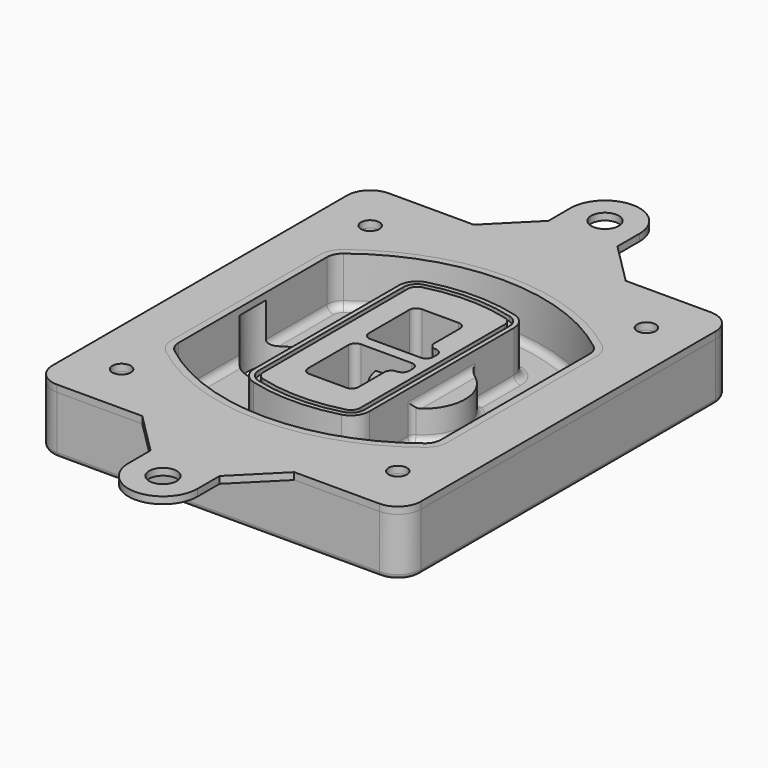
from build123d import *

# Parameters (mm, degrees)
F0_R      = 4
F1_DEPTH  = 25
F2_DEPTH  = 3
F3_DEPTH  = 18
F5_DEPTH  = 21
F6_DEPTH  = 2
F8_DEPTH  = 20
F9_DEPTH  = 16
F10_DEPTH = 25
F7_R      = 6
F7_R_2    = 4
F11_DEPTH = 6
F13_DEPTH = 9
F14_R     = 3
F15_R     = 2
F16_R     = 6
F16_R_2   = 4
F17_DEPTH = 3


# Not quite as in the source:
# - a feature names something its author has since deleted; it is built from what else it names


with BuildPart() as f1:
    # F0 (on Top) → F1 (new body)
    with BuildSketch(Plane.XY):
        with BuildLine():
            ThreePointArc((-80, -80), (-77.0710678119, -87.0710678119), (-70, -90))
            Line((-70, -90), (70, -90))
            ThreePointArc((70, -90), (77.0710678119, -87.0710678119), (80, -80))
            Line((80, -80), (80, 80))
            ThreePointArc((80, 80), (77.0710678119, 87.0710678119), (70, 90))
            Line((70, 90), (-70, 90))
            ThreePointArc((-70, 90), (-77.0710678119, 87.0710678119), (-80, 80))
            Line((-80, 80), (-80, -80))
        make_face()
        with Locations((-60, -67.5)):
            Circle(F0_R, mode=Mode.SUBTRACT)
        with Locations((60, -67.5)):
            Circle(F0_R, mode=Mode.SUBTRACT)
        with Locations((-60, 67.5)):
            Circle(F0_R, mode=Mode.SUBTRACT)
        with BuildLine():
            ThreePointArc((-64, 40.2934422872), (-62.5820384798, 46.4328484224), (-58.6153846154, 51.3286200352))
            ThreePointArc((-58.6153846154, 51.3286200352), (0, 71.5), (58.6153846154, 51.3286200352))
            ThreePointArc((58.6153846154, 51.3286200352), (62.5820384798, 46.4328484224), (64, 40.2934422872))
            Line((64, 40.2934422872), (64, -40.2934422872))
            ThreePointArc((64, -40.2934422872), (62.5820384798, -46.4328484224), (58.6153846154, -51.3286200352))
            ThreePointArc((58.6153846154, -51.3286200352), (0, -71.5), (-58.6153846154, -51.3286200352))
            ThreePointArc((-58.6153846154, -51.3286200352), (-62.5820384798, -46.4328484224), (-64, -40.2934422872))
            Line((-64, -40.2934422872), (-64, 40.2934422872))
        make_face(mode=Mode.SUBTRACT)
        with Locations((60, 67.5)):
            Circle(F0_R, mode=Mode.SUBTRACT)
        with BuildLine():
            ThreePointArc((58.6153846154, 51.3286200352), (0, 71.5), (-58.6153846154, 51.3286200352))
            ThreePointArc((-58.6153846154, 51.3286200352), (-62.5820384798, 46.4328484224), (-64, 40.2934422872))
            Line((-64, 40.2934422872), (-64, -40.2934422872))
            ThreePointArc((-64, -40.2934422872), (-62.5820384798, -46.4328484224), (-58.6153846154, -51.3286200352))
            ThreePointArc((-58.6153846154, -51.3286200352), (0, -71.5), (58.6153846154, -51.3286200352))
            ThreePointArc((58.6153846154, -51.3286200352), (62.5820384798, -46.4328484224), (64, -40.2934422872))
            Line((64, -40.2934422872), (64, 40.2934422872))
            ThreePointArc((64, 40.2934422872), (62.5820384798, 46.4328484224), (58.6153846154, 51.3286200352))
        make_face()
        with BuildLine():
            Line((-60, -40.2934422872), (-60, 40.2934422872))
            ThreePointArc((-60, 40.2934422872), (-58.9871703427, 44.6787323838), (-56.1538461538, 48.1757121072))
            ThreePointArc((-56.1538461538, 48.1757121072), (0, 67.5), (56.1538461538, 48.1757121072))
            ThreePointArc((56.1538461538, 48.1757121072), (58.9871703427, 44.6787323838), (60, 40.2934422872))
            Line((60, 40.2934422872), (60, -40.2934422872))
            ThreePointArc((60, -40.2934422872), (58.9871703427, -44.6787323838), (56.1538461538, -48.1757121072))
            ThreePointArc((56.1538461538, -48.1757121072), (0, -67.5), (-56.1538461538, -48.1757121072))
            ThreePointArc((-56.1538461538, -48.1757121072), (-58.9871703427, -44.6787323838), (-60, -40.2934422872))
        make_face(mode=Mode.SUBTRACT)
        with BuildLine():
            ThreePointArc((-56.1538461538, 48.1757121072), (-58.9871703427, 44.6787323838), (-60, 40.2934422872))
            Line((-60, 40.2934422872), (-60, -40.2934422872))
            ThreePointArc((-60, -40.2934422872), (-58.9871703427, -44.6787323838), (-56.1538461538, -48.1757121072))
            ThreePointArc((-56.1538461538, -48.1757121072), (0, -67.5), (56.1538461538, -48.1757121072))
            ThreePointArc((56.1538461538, -48.1757121072), (58.9871703427, -44.6787323838), (60, -40.2934422872))
            Line((60, -40.2934422872), (60, 40.2934422872))
            ThreePointArc((60, 40.2934422872), (58.9871703427, 44.6787323838), (56.1538461538, 48.1757121072))
            ThreePointArc((56.1538461538, 48.1757121072), (0, 67.5), (-56.1538461538, 48.1757121072))
        make_face()
        with BuildLine():
            ThreePointArc((54.3076923077, 45.8110311612), (56.2910192399, 43.3631453548), (57, 40.2934422872))
            Line((57, 40.2934422872), (57, -40.2934422872))
            ThreePointArc((57, -40.2934422872), (56.2910192399, -43.3631453548), (54.3076923077, -45.8110311612))
            ThreePointArc((54.3076923077, -45.8110311612), (0, -64.5), (-54.3076923077, -45.8110311612))
            ThreePointArc((-54.3076923077, -45.8110311612), (-56.2910192399, -43.3631453548), (-57, -40.2934422872))
            Line((-57, -40.2934422872), (-57, 40.2934422872))
            ThreePointArc((-57, 40.2934422872), (-56.2910192399, 43.3631453548), (-54.3076923077, 45.8110311612))
            ThreePointArc((-54.3076923077, 45.8110311612), (0, 64.5), (54.3076923077, 45.8110311612))
        make_face(mode=Mode.SUBTRACT)
        with BuildLine():
            Line((57, -40.2934422872), (57, 40.2934422872))
            ThreePointArc((57, 40.2934422872), (56.2910192399, 43.3631453548), (54.3076923077, 45.8110311612))
            ThreePointArc((54.3076923077, 45.8110311612), (0, 64.5), (-54.3076923077, 45.8110311612))
            ThreePointArc((-54.3076923077, 45.8110311612), (-56.2910192399, 43.3631453548), (-57, 40.2934422872))
            Line((-57, 40.2934422872), (-57, -40.2934422872))
            ThreePointArc((-57, -40.2934422872), (-56.2910192399, -43.3631453548), (-54.3076923077, -45.8110311612))
            ThreePointArc((-54.3076923077, -45.8110311612), (0, -64.5), (54.3076923077, -45.8110311612))
            ThreePointArc((54.3076923077, -45.8110311612), (56.2910192399, -43.3631453548), (57, -40.2934422872))
        make_face()
    extrude(amount=-F1_DEPTH)

    # F0 (on Top) → F2 (join)
    with BuildSketch(Plane.XY):
        with BuildLine():
            ThreePointArc((-56.1538461538, 48.1757121072), (-58.9871703427, 44.6787323838), (-60, 40.2934422872))
            Line((-60, 40.2934422872), (-60, -40.2934422872))
            ThreePointArc((-60, -40.2934422872), (-58.9871703427, -44.6787323838), (-56.1538461538, -48.1757121072))
            ThreePointArc((-56.1538461538, -48.1757121072), (0, -67.5), (56.1538461538, -48.1757121072))
            ThreePointArc((56.1538461538, -48.1757121072), (58.9871703427, -44.6787323838), (60, -40.2934422872))
            Line((60, -40.2934422872), (60, 40.2934422872))
            ThreePointArc((60, 40.2934422872), (58.9871703427, 44.6787323838), (56.1538461538, 48.1757121072))
            ThreePointArc((56.1538461538, 48.1757121072), (0, 67.5), (-56.1538461538, 48.1757121072))
        make_face()
        with BuildLine():
            ThreePointArc((54.3076923077, 45.8110311612), (56.2910192399, 43.3631453548), (57, 40.2934422872))
            Line((57, 40.2934422872), (57, -40.2934422872))
            ThreePointArc((57, -40.2934422872), (56.2910192399, -43.3631453548), (54.3076923077, -45.8110311612))
            ThreePointArc((54.3076923077, -45.8110311612), (0, -64.5), (-54.3076923077, -45.8110311612))
            ThreePointArc((-54.3076923077, -45.8110311612), (-56.2910192399, -43.3631453548), (-57, -40.2934422872))
            Line((-57, -40.2934422872), (-57, 40.2934422872))
            ThreePointArc((-57, 40.2934422872), (-56.2910192399, 43.3631453548), (-54.3076923077, 45.8110311612))
            ThreePointArc((-54.3076923077, 45.8110311612), (0, 64.5), (54.3076923077, 45.8110311612))
        make_face(mode=Mode.SUBTRACT)
    extrude(amount=F2_DEPTH)

    # F0 (on Top) → F3 (cut)
    with BuildSketch(Plane.XY):
        with BuildLine():
            Line((57, -40.2934422872), (57, 40.2934422872))
            ThreePointArc((57, 40.2934422872), (56.2910192399, 43.3631453548), (54.3076923077, 45.8110311612))
            ThreePointArc((54.3076923077, 45.8110311612), (0, 64.5), (-54.3076923077, 45.8110311612))
            ThreePointArc((-54.3076923077, 45.8110311612), (-56.2910192399, 43.3631453548), (-57, 40.2934422872))
            Line((-57, 40.2934422872), (-57, -40.2934422872))
            ThreePointArc((-57, -40.2934422872), (-56.2910192399, -43.3631453548), (-54.3076923077, -45.8110311612))
            ThreePointArc((-54.3076923077, -45.8110311612), (0, -64.5), (54.3076923077, -45.8110311612))
            ThreePointArc((54.3076923077, -45.8110311612), (56.2910192399, -43.3631453548), (57, -40.2934422872))
        make_face()
    extrude(amount=-F3_DEPTH, mode=Mode.SUBTRACT)

    # F4 (on face) → F5 (join, through all)
    with BuildSketch(Plane.XY.offset(3)):
        with BuildLine():
            ThreePointArc((-25, -39.2465276821), (-23.3511545998, -44.1109737193), (-19.0842911877, -46.9702398883))
            ThreePointArc((-19.0842911877, -46.9702398883), (0, -49.5), (19.0842911877, -46.9702398883))
            ThreePointArc((19.0842911877, -46.9702398883), (23.3511545998, -44.1109737193), (25, -39.2465276821))
            Line((25, -39.2465276821), (25, 39.2465276821))
            ThreePointArc((25, 39.2465276821), (23.3511545998, 44.1109737193), (19.0842911877, 46.9702398883))
            ThreePointArc((19.0842911877, 46.9702398883), (0, 49.5), (-19.0842911877, 46.9702398883))
            ThreePointArc((-19.0842911877, 46.9702398883), (-23.3511545998, 44.1109737193), (-25, 39.2465276821))
            Line((-25, 39.2465276821), (-25, -39.2465276821))
        make_face()
        with BuildLine():
            ThreePointArc((18.5632183908, 45.0393118368), (21.7633659499, 42.89486221), (23, 39.2465276821))
            Line((23, 39.2465276821), (23, -39.2465276821))
            ThreePointArc((23, -39.2465276821), (21.7633659499, -42.89486221), (18.5632183908, -45.0393118368))
            ThreePointArc((18.5632183908, -45.0393118368), (0, -47.5), (-18.5632183908, -45.0393118368))
            ThreePointArc((-18.5632183908, -45.0393118368), (-21.7633659499, -42.89486221), (-23, -39.2465276821))
            Line((-23, -39.2465276821), (-23, 39.2465276821))
            ThreePointArc((-23, 39.2465276821), (-21.7633659499, 42.89486221), (-18.5632183908, 45.0393118368))
            ThreePointArc((-18.5632183908, 45.0393118368), (0, 47.5), (18.5632183908, 45.0393118368))
        make_face(mode=Mode.SUBTRACT)
        with BuildLine():
            Line((23, -39.2465276821), (23, 39.2465276821))
            ThreePointArc((23, 39.2465276821), (21.7633659499, 42.89486221), (18.5632183908, 45.0393118368))
            ThreePointArc((18.5632183908, 45.0393118368), (0, 47.5), (-18.5632183908, 45.0393118368))
            ThreePointArc((-18.5632183908, 45.0393118368), (-21.7633659499, 42.89486221), (-23, 39.2465276821))
            Line((-23, 39.2465276821), (-23, -39.2465276821))
            ThreePointArc((-23, -39.2465276821), (-21.7633659499, -42.89486221), (-18.5632183908, -45.0393118368))
            ThreePointArc((-18.5632183908, -45.0393118368), (0, -47.5), (18.5632183908, -45.0393118368))
            ThreePointArc((18.5632183908, -45.0393118368), (21.7633659499, -42.89486221), (23, -39.2465276821))
        make_face()
        with BuildLine():
            ThreePointArc((18.0421455939, 43.1083837852), (20.1755772999, 41.6787507007), (21, 39.2465276821))
            Line((21, 39.2465276821), (21, -39.2465276821))
            ThreePointArc((21, -39.2465276821), (20.1755772999, -41.6787507007), (18.0421455939, -43.1083837852))
            ThreePointArc((18.0421455939, -43.1083837852), (0, -45.5), (-18.0421455939, -43.1083837852))
            ThreePointArc((-18.0421455939, -43.1083837852), (-20.1755772999, -41.6787507007), (-21, -39.2465276821))
            Line((-21, -39.2465276821), (-21, 39.2465276821))
            ThreePointArc((-21, 39.2465276821), (-20.1755772999, 41.6787507007), (-18.0421455939, 43.1083837852))
            ThreePointArc((-18.0421455939, 43.1083837852), (0, 45.5), (18.0421455939, 43.1083837852))
        make_face(mode=Mode.SUBTRACT)
        with BuildLine():
            Line((21, -39.2465276821), (21, 39.2465276821))
            ThreePointArc((21, 39.2465276821), (20.1755772999, 41.6787507007), (18.0421455939, 43.1083837852))
            ThreePointArc((18.0421455939, 43.1083837852), (0, 45.5), (-18.0421455939, 43.1083837852))
            ThreePointArc((-18.0421455939, 43.1083837852), (-20.1755772999, 41.6787507007), (-21, 39.2465276821))
            Line((-21, 39.2465276821), (-21, -39.2465276821))
            ThreePointArc((-21, -39.2465276821), (-20.1755772999, -41.6787507007), (-18.0421455939, -43.1083837852))
            ThreePointArc((-18.0421455939, -43.1083837852), (0, -45.5), (18.0421455939, -43.1083837852))
            ThreePointArc((18.0421455939, -43.1083837852), (20.1755772999, -41.6787507007), (21, -39.2465276821))
        make_face()
        with BuildLine():
            Line((-8, -2.5), (14, -2.5))
            ThreePointArc((14, -2.5), (16.1213203436, -3.3786796564), (17, -5.5))
            Line((17, -5.5), (17, -7.5))
            ThreePointArc((17, -7.5), (16.1213203436, -9.6213203436), (14, -10.5))
            ThreePointArc((14, -10.5), (11.8786796564, -11.3786796564), (11, -13.5))
            Line((11, -13.5), (11, -27.5))
            ThreePointArc((11, -27.5), (10.1213203436, -29.6213203436), (8, -30.5))
            Line((8, -30.5), (-8, -30.5))
            ThreePointArc((-8, -30.5), (-10.1213203436, -29.6213203436), (-11, -27.5))
            Line((-11, -27.5), (-11, -5.5))
            ThreePointArc((-11, -5.5), (-10.1213203436, -3.3786796564), (-8, -2.5))
        make_face(mode=Mode.SUBTRACT)
        with BuildLine():
            ThreePointArc((-8, 2.5), (-10.1213203436, 3.3786796564), (-11, 5.5))
            Line((-11, 5.5), (-11, 27.5))
            ThreePointArc((-11, 27.5), (-10.1213203436, 29.6213203436), (-8, 30.5))
            Line((-8, 30.5), (8, 30.5))
            ThreePointArc((8, 30.5), (10.1213203436, 29.6213203436), (11, 27.5))
            Line((11, 27.5), (11, 13.5))
            ThreePointArc((11, 13.5), (11.8786796564, 11.3786796564), (14, 10.5))
            ThreePointArc((14, 10.5), (16.1213203436, 9.6213203436), (17, 7.5))
            Line((17, 7.5), (17, 5.5))
            ThreePointArc((17, 5.5), (16.1213203436, 3.3786796564), (14, 2.5))
            Line((14, 2.5), (-8, 2.5))
        make_face(mode=Mode.SUBTRACT)
    extrude(amount=-F5_DEPTH)

    # F4 (on face) → F6 (cut)
    with BuildSketch(Plane.XY.offset(3)):
        with BuildLine():
            Line((23, -39.2465276821), (23, 39.2465276821))
            ThreePointArc((23, 39.2465276821), (21.7633659499, 42.89486221), (18.5632183908, 45.0393118368))
            ThreePointArc((18.5632183908, 45.0393118368), (0, 47.5), (-18.5632183908, 45.0393118368))
            ThreePointArc((-18.5632183908, 45.0393118368), (-21.7633659499, 42.89486221), (-23, 39.2465276821))
            Line((-23, 39.2465276821), (-23, -39.2465276821))
            ThreePointArc((-23, -39.2465276821), (-21.7633659499, -42.89486221), (-18.5632183908, -45.0393118368))
            ThreePointArc((-18.5632183908, -45.0393118368), (0, -47.5), (18.5632183908, -45.0393118368))
            ThreePointArc((18.5632183908, -45.0393118368), (21.7633659499, -42.89486221), (23, -39.2465276821))
        make_face()
        with BuildLine():
            ThreePointArc((18.0421455939, 43.1083837852), (20.1755772999, 41.6787507007), (21, 39.2465276821))
            Line((21, 39.2465276821), (21, -39.2465276821))
            ThreePointArc((21, -39.2465276821), (20.1755772999, -41.6787507007), (18.0421455939, -43.1083837852))
            ThreePointArc((18.0421455939, -43.1083837852), (0, -45.5), (-18.0421455939, -43.1083837852))
            ThreePointArc((-18.0421455939, -43.1083837852), (-20.1755772999, -41.6787507007), (-21, -39.2465276821))
            Line((-21, -39.2465276821), (-21, 39.2465276821))
            ThreePointArc((-21, 39.2465276821), (-20.1755772999, 41.6787507007), (-18.0421455939, 43.1083837852))
            ThreePointArc((-18.0421455939, 43.1083837852), (0, 45.5), (18.0421455939, 43.1083837852))
        make_face(mode=Mode.SUBTRACT)
    extrude(amount=-F6_DEPTH, mode=Mode.SUBTRACT)

    # F7 (on face) → F8 (join)
    with BuildSketch(Plane(origin=(0, 0, -25), x_dir=(1, 0, 0), z_dir=(0, 0, -1))):
        with BuildLine():
            ThreePointArc((3.28842436, 0), (16.7567035675, 13.4682792075), (30.224982775, 0))
            Line((30.224982775, 0), (35.224982775, 0))
            ThreePointArc((35.224982775, 0), (16.7567035675, 18.4682792075), (-1.71157564, 0))
            Line((-1.71157564, 0), (3.28842436, 0))
        make_face()
        with BuildLine():
            Line((3.28842436, 0), (30.224982775, 0))
            ThreePointArc((30.224982775, 0), (16.7567035675, 13.4682792075), (3.28842436, 0))
        make_face()
        with BuildLine():
            ThreePointArc((3.28842436, 0), (16.7567035675, -13.4682792075), (30.224982775, 0))
            Line((30.224982775, 0), (3.28842436, 0))
        make_face()
        with BuildLine():
            Line((35.224982775, 0), (30.224982775, 0))
            ThreePointArc((30.224982775, 0), (16.7567035675, -13.4682792075), (3.28842436, 0))
            Line((3.28842436, 0), (-1.71157564, 0))
            ThreePointArc((-1.71157564, 0), (16.7567035675, -18.4682792075), (35.224982775, 0))
        make_face()
    extrude(amount=-F8_DEPTH)

    # F7 (on face) → F9 (cut)
    with BuildSketch(Plane(origin=(0, 0, -25), x_dir=(1, 0, 0), z_dir=(0, 0, -1))):
        with BuildLine():
            Line((3.28842436, 0), (30.224982775, 0))
            ThreePointArc((30.224982775, 0), (16.7567035675, 13.4682792075), (3.28842436, 0))
        make_face()
        with BuildLine():
            ThreePointArc((3.28842436, 0), (16.7567035675, -13.4682792075), (30.224982775, 0))
            Line((30.224982775, 0), (3.28842436, 0))
        make_face()
    extrude(amount=-F9_DEPTH, mode=Mode.SUBTRACT)

    # F7 (on face) → F10 (cut)
    with BuildSketch(Plane(origin=(0, 0, -25), x_dir=(1, 0, 0), z_dir=(0, 0, -1))):
        with BuildLine():
            Line((-59.0318229325, 0), (-32.0952645175, 0))
            ThreePointArc((-32.0952645175, 0), (-45.563543725, 13.4682792075), (-59.0318229325, 0))
        make_face()
        with BuildLine():
            ThreePointArc((-59.0318229325, 0), (-45.563543725, -13.4682792075), (-32.0952645175, 0))
            Line((-32.0952645175, 0), (-59.0318229325, 0))
        make_face()
    extrude(amount=-F10_DEPTH, mode=Mode.SUBTRACT)

    # F7 (on face) → F11 (cut)
    with BuildSketch(Plane(origin=(0, 0, -25), x_dir=(1, 0, 0), z_dir=(0, 0, -1))):
        with Locations((60, -67.5)):
            Circle(F7_R)
        with Locations((60, -67.5)):
            Circle(F7_R_2, mode=Mode.SUBTRACT)
        with Locations((-60, -67.5)):
            Circle(F7_R)
        with Locations((-60, -67.5)):
            Circle(F7_R_2, mode=Mode.SUBTRACT)
        with Locations((-60, 67.5)):
            Circle(F7_R)
        with Locations((-60, 67.5)):
            Circle(F7_R_2, mode=Mode.SUBTRACT)
        with Locations((60, 67.5)):
            Circle(F7_R)
        with Locations((60, 67.5)):
            Circle(F7_R_2, mode=Mode.SUBTRACT)
    extrude(amount=-F11_DEPTH, mode=Mode.SUBTRACT)

    # F12 (on face) → F13 (cut, through all)
    with BuildSketch(Plane(origin=(0, 0, -9), x_dir=(1, 0, 0), z_dir=(0, 0, -1))):
        with BuildLine():
            Line((11, 13.5), (11, 17.5481537753))
            ThreePointArc((11, 17.5481537753), (2.5696536419, 11.8239143813), (-1.5415842455, 2.5))
            Line((-1.5415842455, 2.5), (3.5224848595, 2.5))
            ThreePointArc((3.5224848595, 2.5), (6.1857188154, 8.3455872281), (11.2536447004, 12.2927168648))
            ThreePointArc((11.2536447004, 12.2927168648), (11.0640958889, 12.8831798879), (11, 13.5))
        make_face()
        with BuildLine():
            ThreePointArc((11.2536447004, -12.2927168648), (6.1857188154, -8.3455872281), (3.5224848595, -2.5))
            Line((3.5224848595, -2.5), (-1.5415842455, -2.5))
            ThreePointArc((-1.5415842455, -2.5), (2.5696536419, -11.8239143813), (11, -17.5481537753))
            Line((11, -17.5481537753), (11, -13.5))
            ThreePointArc((11, -13.5), (11.0640958889, -12.8831798879), (11.2536447004, -12.2927168648))
        make_face()
        with BuildLine():
            ThreePointArc((11.2536447004, 12.2927168648), (6.1857188154, 8.3455872281), (3.5224848595, 2.5))
            Line((3.5224848595, 2.5), (14, 2.5))
            ThreePointArc((14, 2.5), (16.1213203436, 3.3786796564), (17, 5.5))
            Line((17, 5.5), (17, 7.5))
            ThreePointArc((17, 7.5), (16.1213203436, 9.6213203436), (14, 10.5))
            ThreePointArc((14, 10.5), (12.3601599782, 10.9878446101), (11.2536447004, 12.2927168648))
        make_face()
        with BuildLine():
            Line((14, -2.5), (3.5224848595, -2.5))
            ThreePointArc((3.5224848595, -2.5), (6.1857188154, -8.3455872281), (11.2536447004, -12.2927168648))
            ThreePointArc((11.2536447004, -12.2927168648), (12.3601599782, -10.9878446101), (14, -10.5))
            ThreePointArc((14, -10.5), (16.1213203436, -9.6213203436), (17, -7.5))
            Line((17, -7.5), (17, -5.5))
            ThreePointArc((17, -5.5), (16.1213203436, -3.3786796564), (14, -2.5))
        make_face()
    extrude(amount=F13_DEPTH, mode=Mode.SUBTRACT)

    # F14
    f14_edges = [f1.edges().sort_by_distance(p)[0] for p in [
        (-57, -23.703476, -18),
        (-57, 23.703476, -18),
        (25, 0, -5),
        (25, 16.526506, -11.5),
        (25, -16.526506, -11.5),
        (25, -27.886517, -18),
        (35.224983, 0, -18),
    ]]
    fillet(f14_edges, radius=F14_R)

    # F15
    f15_edges = [f1.edges().sort_by_distance(p)[0] for p in [
        (0, -90, -25),
    ]]
    fillet(f15_edges, radius=F15_R)


with BuildPart() as f17:
    # F16 (on face) → F17 (new body, through all)
    with BuildSketch(Plane.XY):
        with BuildLine():
            Line((33, -90), (-33, -90))
            Line((-33, -90), (-15, -108))
            Line((-15, -108), (-15, -120))
            ThreePointArc((-15, -120), (0, -135), (15, -120))
            Line((15, -120), (15, -108))
            Line((15, -108), (33, -90))
        make_face()
        with Locations((0, -120)):
            Circle(F16_R, mode=Mode.SUBTRACT)
        with BuildLine():
            Line((-15, 108), (-33, 90))
            Line((-33, 90), (33, 90))
            Line((33, 90), (15, 108))
            Line((15, 108), (15, 120))
            ThreePointArc((15, 120), (0, 135), (-15, 120))
            Line((-15, 120), (-15, 108))
        make_face()
        with Locations((0, 120)):
            Circle(F16_R, mode=Mode.SUBTRACT)
        with BuildLine():
            Line((33, 90), (-33, 90))
            Line((-33, 90), (-70, 90))
            ThreePointArc((-70, 90), (-77.0710678119, 87.0710678119), (-80, 80))
            Line((-80, 80), (-80, -80))
            ThreePointArc((-80, -80), (-77.0710678119, -87.0710678119), (-70, -90))
            Line((-70, -90), (-33, -90))
            Line((-33, -90), (33, -90))
            Line((33, -90), (70, -90))
            ThreePointArc((70, -90), (77.0710678119, -87.0710678119), (80, -80))
            Line((80, -80), (80, 80))
            ThreePointArc((80, 80), (77.0710678119, 87.0710678119), (70, 90))
            Line((70, 90), (33, 90))
        make_face()
        with Locations((-60, -67.5)):
            Circle(F16_R_2, mode=Mode.SUBTRACT)
        with Locations((60, -67.5)):
            Circle(F16_R_2, mode=Mode.SUBTRACT)
        with Locations((-60, 67.5)):
            Circle(F16_R_2, mode=Mode.SUBTRACT)
        with BuildLine():
            ThreePointArc((-60, 40.2934422872), (-58.9871703427, 44.6787323838), (-56.1538461538, 48.1757121072))
            ThreePointArc((-56.1538461538, 48.1757121072), (0, 67.5), (56.1538461538, 48.1757121072))
            ThreePointArc((56.1538461538, 48.1757121072), (58.9871703427, 44.6787323838), (60, 40.2934422872))
            Line((60, 40.2934422872), (60, -40.2934422872))
            ThreePointArc((60, -40.2934422872), (58.9871703427, -44.6787323838), (56.1538461538, -48.1757121072))
            ThreePointArc((56.1538461538, -48.1757121072), (0, -67.5), (-56.1538461538, -48.1757121072))
            ThreePointArc((-56.1538461538, -48.1757121072), (-58.9871703427, -44.6787323838), (-60, -40.2934422872))
            Line((-60, -40.2934422872), (-60, 40.2934422872))
        make_face(mode=Mode.SUBTRACT)
        with Locations((60, 67.5)):
            Circle(F16_R_2, mode=Mode.SUBTRACT)
    extrude(amount=F17_DEPTH)


solid = Compound([f1.part, f17.part])
